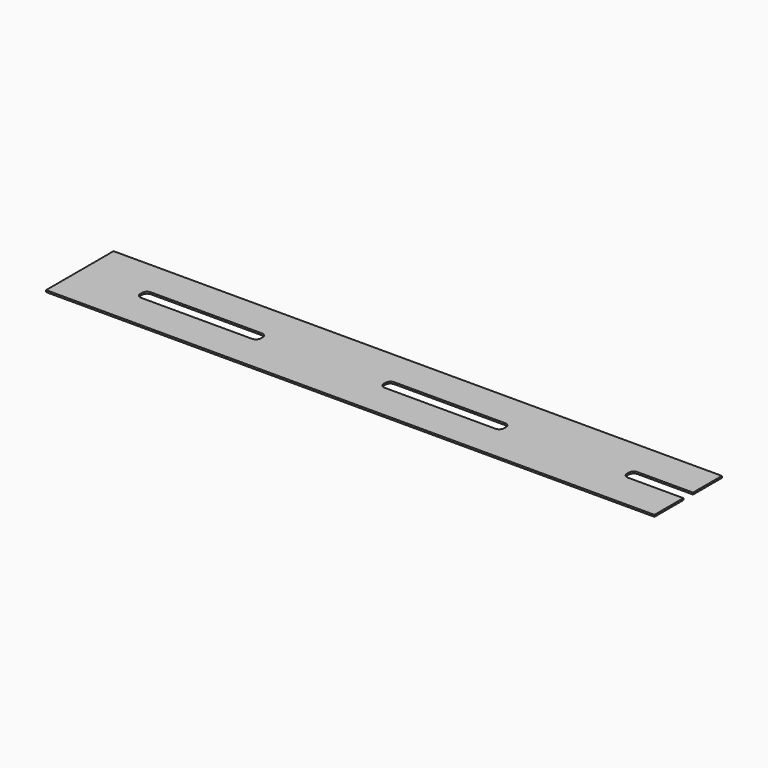
from build123d import *

# Parameters (mm, degrees)
F1_DEPTH = 0.15


# Not quite as in the source:
# - a feature names something its author has since deleted; it is built from what else it names


with BuildPart() as f1:
    # F0 (on Top) → F1 (new body)
    with BuildSketch(Plane.XY):
        with BuildLine():
            Line((10.1, -0.5), (10.1, -3.5))
            Line((10.1, -3.5), (20.2, -3.5))
            Line((20.2, -3.5), (30.3, -3.5))
            Line((30.3, -3.5), (30.3, -0.5))
            Line((30.3, -0.5), (25.7, -0.5))
            ThreePointArc((25.7, -0.5), (25.4171572875, -0.3828427125), (25.3, -0.1))
            Line((25.3, -0.1), (25.3, 0.1))
            ThreePointArc((25.3, 0.1), (25.4171572875, 0.3828427125), (25.7, 0.5))
            Line((25.7, 0.5), (30.3, 0.5))
            Line((30.3, 0.5), (30.3, 3.5))
            Line((30.3, 3.5), (20.2, 3.5))
            Line((20.2, 3.5), (10.1, 3.5))
            Line((10.1, 3.5), (10.1, 0.5))
            Line((10.1, 0.5), (14.7, 0.5))
            ThreePointArc((14.7, 0.5), (14.9828427125, 0.3828427125), (15.1, 0.1))
            Line((15.1, 0.1), (15.1, -0.1))
            ThreePointArc((15.1, -0.1), (14.9828427125, -0.3828427125), (14.7, -0.5))
            Line((14.7, -0.5), (10.1, -0.5))
        make_face()
        with BuildLine():
            Line((30.3, -0.5), (30.3, -3.5))
            Line((30.3, -3.5), (40.4, -3.5))
            Line((40.4, -3.5), (50.5, -3.5))
            Line((50.5, -3.5), (50.5, -0.5))
            Line((50.5, -0.5), (45.9, -0.5))
            ThreePointArc((45.9, -0.5), (45.6171572875, -0.3828427125), (45.5, -0.1))
            Line((45.5, -0.1), (45.5, 0.1))
            ThreePointArc((45.5, 0.1), (45.6171572875, 0.3828427125), (45.9, 0.5))
            Line((45.9, 0.5), (50.5, 0.5))
            Line((50.5, 0.5), (50.5, 3.5))
            Line((50.5, 3.5), (40.4, 3.5))
            Line((40.4, 3.5), (30.3, 3.5))
            Line((30.3, 3.5), (30.3, 0.5))
            Line((30.3, 0.5), (34.9, 0.5))
            ThreePointArc((34.9, 0.5), (35.1828427125, 0.3828427125), (35.3, 0.1))
            Line((35.3, 0.1), (35.3, -0.1))
            ThreePointArc((35.3, -0.1), (35.1828427125, -0.3828427125), (34.9, -0.5))
            Line((34.9, -0.5), (30.3, -0.5))
        make_face()
        with BuildLine():
            Line((0, 3.5), (0, -3.5))
            Line((0, -3.5), (10.1, -3.5))
            Line((10.1, -3.5), (10.1, -0.5))
            Line((10.1, -0.5), (5.5, -0.5))
            ThreePointArc((5.5, -0.5), (5.2171572875, -0.3828427125), (5.1, -0.1))
            Line((5.1, -0.1), (5.1, 0.1))
            ThreePointArc((5.1, 0.1), (5.2171572875, 0.3828427125), (5.5, 0.5))
            Line((5.5, 0.5), (10.1, 0.5))
            Line((10.1, 0.5), (10.1, 3.5))
            Line((10.1, 3.5), (0, 3.5))
        make_face()
    extrude(amount=F1_DEPTH)


solid = f1.part
